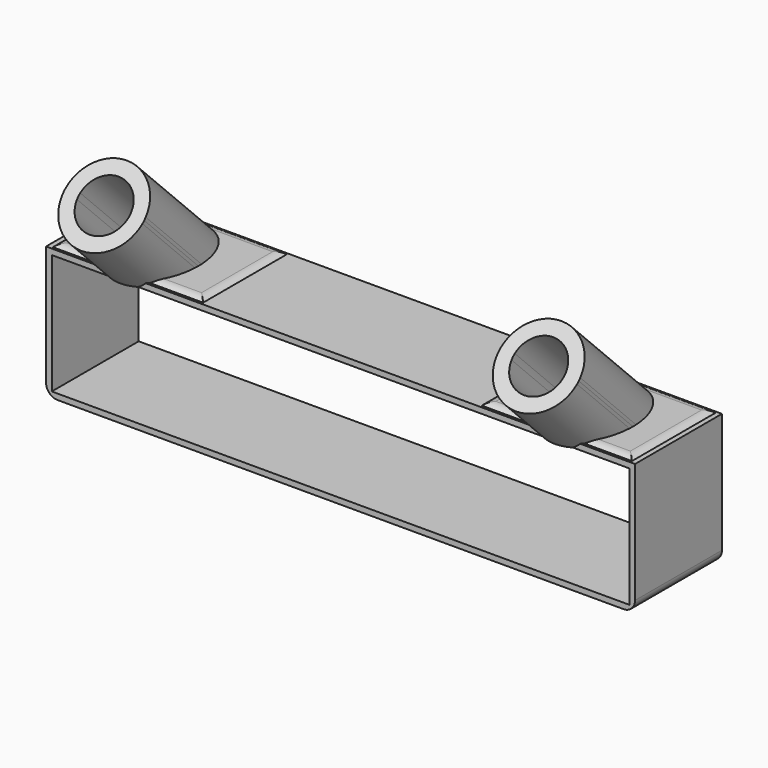
from build123d import *

# Parameters (mm, degrees)
F1_DEPTH       = 25
F2_ANGLE       = 45
F3_W           = 19
F3_H           = 1
F4_DEPTH       = 51
F4_DEPTH_BACK  = 51
F5_DEPTH       = 24
F5_DEPTH_BACK  = 24
F6_W           = 103
F6_H           = 23
F6_W_2         = 101
F6_H_2         = 21
F7_DEPTH       = 13.5
F7_DEPTH_BACK  = 5.5
F8_DEPTH       = 25
F8_DEPTH_BACK  = 25
F9_T1_DEPTH    = 35.6602540378
F9_T3_DEPTH    = 27.6602540378
F9_S1_T1_DEPTH = 35.6602540378
F9_S1_T3_DEPTH = 27.6602540378
F10_R          = 2


# Not quite as in the source:
# - a fillet or chamfer that OpenCascade refuses, or shapes differently, is made with other operations: its cross-section is extruded or revolved along the edge and cut away or added


with BuildPart() as f1:
    # F0 (on Front) → F1 (new body)
    with BuildSketch(Plane.XZ):
        with BuildLine():
            Line((-33.527864045, 22.0619773716), (-31.0178799781, 22.0619773716))
            ThreePointArc((-31.0178799781, 22.0619773716), (-38, 28.5619773716), (-44.9821200219, 22.0619773716))
            Line((-44.9821200219, 22.0619773716), (-42.472135955, 22.0619773716))
            ThreePointArc((-42.472135955, 22.0619773716), (-38, 26.0619773716), (-33.527864045, 22.0619773716))
        make_face()
        with BuildLine():
            Line((-42.472135955, 22.0619773716), (-44.9821200219, 22.0619773716))
            ThreePointArc((-44.9821200219, 22.0619773716), (-45, 21.5619773716), (-44.9821200219, 21.0619773716))
            Line((-44.9821200219, 21.0619773716), (-42.472135955, 21.0619773716))
            ThreePointArc((-42.472135955, 21.0619773716), (-42.5, 21.5619773716), (-42.472135955, 22.0619773716))
        make_face()
        with BuildLine():
            ThreePointArc((-44.9821200219, 21.0619773716), (-38, 14.5619773716), (-31.0178799781, 21.0619773716))
            Line((-31.0178799781, 21.0619773716), (-33.527864045, 21.0619773716))
            ThreePointArc((-33.527864045, 21.0619773716), (-38, 17.0619773716), (-42.472135955, 21.0619773716))
            Line((-42.472135955, 21.0619773716), (-44.9821200219, 21.0619773716))
        make_face()
        with BuildLine():
            ThreePointArc((-31.0178799781, 21.0619773716), (-31.0044714226, 21.3118175758), (-31, 21.5619773716))
            ThreePointArc((-31, 21.5619773716), (-31.0044714226, 21.8121371673), (-31.0178799781, 22.0619773716))
            Line((-31.0178799781, 22.0619773716), (-33.527864045, 22.0619773716))
            ThreePointArc((-33.527864045, 22.0619773716), (-33.5069714113, 21.8123652731), (-33.5, 21.5619773716))
            ThreePointArc((-33.5, 21.5619773716), (-33.5069714113, 21.31158947), (-33.527864045, 21.0619773716))
            Line((-33.527864045, 21.0619773716), (-31.0178799781, 21.0619773716))
        make_face()
    extrude(amount=F1_DEPTH)


with BuildPart() as f1b:
    # F0 (on Front) → F1, piece 2 (new body)
    with BuildSketch(Plane.XZ):
        with BuildLine():
            ThreePointArc((44.9821200219, 22.0619773716), (38, 28.5619773716), (31.0178799781, 22.0619773716))
            Line((31.0178799781, 22.0619773716), (33.527864045, 22.0619773716))
            ThreePointArc((33.527864045, 22.0619773716), (38, 26.0619773716), (42.472135955, 22.0619773716))
            Line((42.472135955, 22.0619773716), (44.9821200219, 22.0619773716))
        make_face()
        with BuildLine():
            Line((33.527864045, 22.0619773716), (31.0178799781, 22.0619773716))
            ThreePointArc((31.0178799781, 22.0619773716), (31, 21.5619773716), (31.0178799781, 21.0619773716))
            Line((31.0178799781, 21.0619773716), (33.527864045, 21.0619773716))
            ThreePointArc((33.527864045, 21.0619773716), (33.5, 21.5619773716), (33.527864045, 22.0619773716))
        make_face()
        with BuildLine():
            Line((33.527864045, 21.0619773716), (31.0178799781, 21.0619773716))
            ThreePointArc((31.0178799781, 21.0619773716), (38, 14.5619773716), (44.9821200219, 21.0619773716))
            Line((44.9821200219, 21.0619773716), (42.472135955, 21.0619773716))
            ThreePointArc((42.472135955, 21.0619773716), (38, 17.0619773716), (33.527864045, 21.0619773716))
        make_face()
        with BuildLine():
            ThreePointArc((45, 21.5619773716), (44.9955285774, 21.8121371673), (44.9821200219, 22.0619773716))
            Line((44.9821200219, 22.0619773716), (42.472135955, 22.0619773716))
            ThreePointArc((42.472135955, 22.0619773716), (42.4930285887, 21.8123652731), (42.5, 21.5619773716))
            ThreePointArc((42.5, 21.5619773716), (42.4930285887, 21.31158947), (42.472135955, 21.0619773716))
            Line((42.472135955, 21.0619773716), (44.9821200219, 21.0619773716))
            ThreePointArc((44.9821200219, 21.0619773716), (44.9955285774, 21.3118175758), (45, 21.5619773716))
        make_face()
    extrude(amount=F1_DEPTH)


with BuildPart() as f1_1:
    # F2: moved
    add(f1.part.rotate(Axis((25, 0, 21.5619773716), (-1, 0, 0)), F2_ANGLE))


with BuildPart() as f1b_1:
    # F2: moved
    add(f1b.part.rotate(Axis((25, 0, 21.5619773716), (-1, 0, 0)), F2_ANGLE))


with BuildPart() as f4:
    # F3 (on Right) → F4 (new body, two sides)
    with BuildSketch(Plane.YZ) as f4_sk:
        with Locations((-3.955035704, 26.910741644)):
            Rectangle(F3_W, F3_H)
    extrude(amount=F4_DEPTH)
    extrude(f4_sk.sketch, amount=-F4_DEPTH_BACK)

    # F3 (on Right) → F5 (cut, two sides)
    with BuildSketch(Plane.YZ) as f5_sk:
        with Locations((-3.955035704, 26.910741644)):
            Rectangle(F3_W, F3_H)
    extrude(amount=-F5_DEPTH, mode=Mode.SUBTRACT)
    extrude(f5_sk.sketch, amount=F5_DEPTH_BACK, mode=Mode.SUBTRACT)

    # F9: fillet of radius 2 on 4 edges, made by hand

    # F9_s2 → F9_t1 (cut)
    with BuildSketch(Plane.YZ.offset(19.6698729811)):
        with BuildLine():
            ThreePointArc((3.8129134884, 27.410741644), (4.8129134884, 27.1427924515), (5.544964296, 26.410741644))
            Line((5.544964296, 26.410741644), (5.544964296, 27.410741644))
            Line((5.544964296, 27.410741644), (3.8129134884, 27.410741644))
        make_face()
        with BuildLine():
            ThreePointArc((-13.455035704, 26.410741644), (-12.7229848965, 27.1427924515), (-11.7229848965, 27.410741644))
            Line((-11.7229848965, 27.410741644), (-13.455035704, 27.410741644))
            Line((-13.455035704, 27.410741644), (-13.455035704, 26.410741644))
        make_face()
    extrude(amount=F9_T1_DEPTH, mode=Mode.SUBTRACT)

    # F9_s4 → F9_t3 (cut)
    with BuildSketch(Plane.XZ.offset(-9.8750913149)):
        with BuildLine():
            ThreePointArc((25.7320508076, 27.410741644), (24.7320508076, 27.1427924515), (24, 26.410741644))
            Line((24, 26.410741644), (24, 27.410741644))
            Line((24, 27.410741644), (25.7320508076, 27.410741644))
        make_face()
        with BuildLine():
            ThreePointArc((49.2679491924, 27.410741644), (50.2679491924, 27.1427924515), (51, 26.410741644))
            Line((51, 26.410741644), (51, 27.410741644))
            Line((51, 27.410741644), (49.2679491924, 27.410741644))
        make_face()
    extrude(amount=F9_T3_DEPTH, mode=Mode.SUBTRACT)

    # F9#s1: fillet of radius 2 on 4 edges, made by hand

    # F9_s1_s2 → F9_s1_t1 (cut)
    with BuildSketch(Plane.YZ.offset(-55.3301270189)):
        with BuildLine():
            ThreePointArc((3.8129134884, 27.410741644), (4.8129134884, 27.1427924515), (5.544964296, 26.410741644))
            Line((5.544964296, 26.410741644), (5.5796053121, 26.430741644))
            ThreePointArc((5.5796053121, 26.430741644), (5.584964296, 26.910741644), (5.584964296, 27.410741644))
            Line((5.584964296, 27.410741644), (5.544964296, 27.450741644))
            Line((5.544964296, 27.450741644), (3.8129134884, 27.450741644))
            Line((3.8129134884, 27.450741644), (3.8129134884, 27.410741644))
        make_face()
        with BuildLine():
            ThreePointArc((-13.455035704, 26.410741644), (-12.7229848965, 27.1427924515), (-11.7229848965, 27.410741644))
            Line((-11.7229848965, 27.410741644), (-11.7229848965, 27.450741644))
            Line((-11.7229848965, 27.450741644), (-13.455035704, 27.450741644))
            Line((-13.455035704, 27.450741644), (-13.495035704, 27.410741644))
            ThreePointArc((-13.495035704, 27.410741644), (-13.495035704, 26.910741644), (-13.4896767202, 26.430741644))
            Line((-13.4896767202, 26.430741644), (-13.455035704, 26.410741644))
        make_face()
    extrude(amount=F9_S1_T1_DEPTH, mode=Mode.SUBTRACT)

    # F9_s1_s4 → F9_s1_t3 (cut)
    with BuildSketch(Plane.XZ.offset(-9.8750913149)):
        with BuildLine():
            ThreePointArc((-49.2679491924, 27.410741644), (-50.2679491924, 27.1427924515), (-51, 26.410741644))
            Line((-51, 26.410741644), (-51.0346410162, 26.430741644))
            ThreePointArc((-51.0346410162, 26.430741644), (-51.04, 26.910741644), (-51.04, 27.410741644))
            Line((-51.04, 27.410741644), (-51, 27.450741644))
            Line((-51, 27.450741644), (-49.2679491924, 27.450741644))
            Line((-49.2679491924, 27.450741644), (-49.2679491924, 27.410741644))
        make_face()
        with BuildLine():
            ThreePointArc((-25.7320508076, 27.410741644), (-24.7320508076, 27.1427924515), (-24, 26.410741644))
            Line((-24, 26.410741644), (-23.9653589838, 26.430741644))
            ThreePointArc((-23.9653589838, 26.430741644), (-23.96, 26.910741644), (-23.96, 27.410741644))
            Line((-23.96, 27.410741644), (-24, 27.450741644))
            Line((-24, 27.450741644), (-25.7320508076, 27.450741644))
            Line((-25.7320508076, 27.450741644), (-25.7320508076, 27.410741644))
        make_face()
    extrude(amount=F9_S1_T3_DEPTH, mode=Mode.SUBTRACT)


with BuildPart() as f7:
    # F6 (on Front) → F7 (new body, two sides)
    with BuildSketch(Plane.XZ) as f7_sk:
        with Locations((0, 15.3747174848)):
            Rectangle(F6_W, F6_H)
        with Locations((0, 15.3747174848)):
            Rectangle(F6_W_2, F6_H_2, mode=Mode.SUBTRACT)
    extrude(amount=F7_DEPTH)
    extrude(f7_sk.sketch, amount=-F7_DEPTH_BACK)

    # F10
    f10_edges = [f7.edges().sort_by_distance(p)[0] for p in [
        (51.5, -4, 3.874717),
        (-51.5, -4, 3.874717),
    ]]
    fillet(f10_edges, radius=F10_R)


with BuildPart() as f8_tool:
    # F6 (on Front) → F8 (new body, two sides)
    with BuildSketch(Plane.XZ) as f8_sk:
        with Locations((0, 15.3747174848)):
            Rectangle(F6_W_2, F6_H_2)
    extrude(amount=F8_DEPTH)
    extrude(f8_sk.sketch, amount=-F8_DEPTH_BACK)


with BuildPart() as f1_2:
    add(f1_1.part)

    # F8: cut by f8_tool
    add(f8_tool.part, mode=Mode.SUBTRACT)


with BuildPart() as f1b_2:
    add(f1b_1.part)

    # F8: cut by f8_tool
    add(f8_tool.part, mode=Mode.SUBTRACT)


solid = Compound([f4.part, f7.part, f1_2.part, f1b_2.part])
